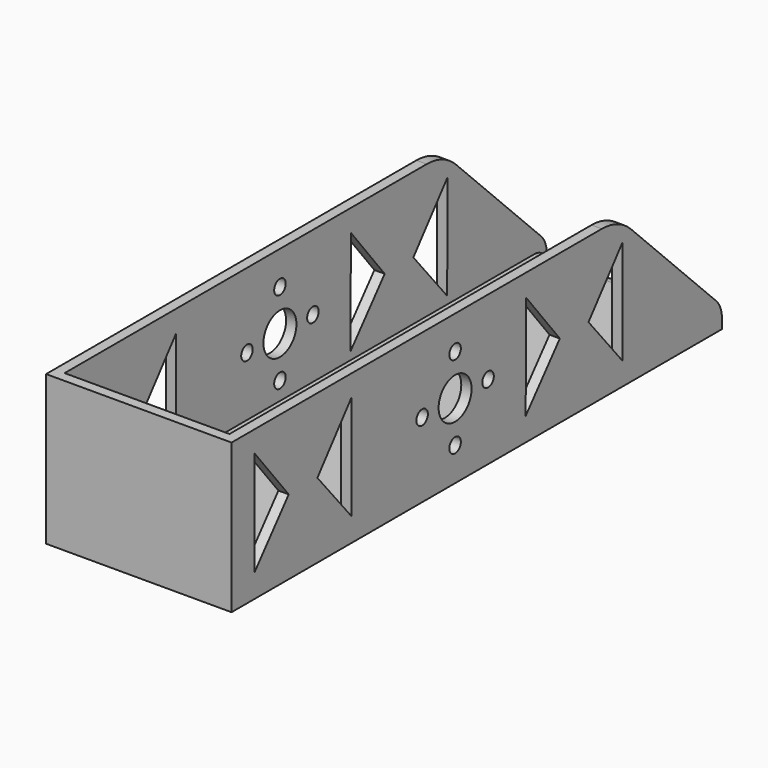
from build123d import *

# Parameters (mm, degrees)
F0_W      = 36
F0_H      = 119
F1_DEPTH  = 3
F3_DEPTH  = 26
F5_SIZE   = 25
F6_R      = 10
F7_R      = 2.99999
F8_R      = 5
F10_DEPTH = 25
F9_R      = 1.4
F9_R_2    = 4
F11_DEPTH = 36.001


# Not quite as in the source:
# - a fillet or chamfer is up to 0.001 mm smaller than in the source, because OpenCascade refuses the exact size


with BuildPart() as f1:
    # F0 (on Top) → F1 (new body)
    with BuildSketch(Plane.XY):
        Rectangle(F0_W, F0_H)
    extrude(amount=F1_DEPTH)

    # F2 (on face) → F3 (join)
    with BuildSketch(Plane.XY.offset(3)):
        Polygon((16, -57.5), (-16, -57.5), (-16, 57.5), (-16, 59.5), (-18, 59.5), (-18, -59.5), (18, -59.5), (18, 59.5), (16, 59.5), (16, 57.5), align=None)
    extrude(amount=F3_DEPTH)

    # F5
    f5_edges = [f1.edges().sort_by_distance(p)[0] for p in [
        (-17, 59.5, 29),
        (17, 59.5, 29),
    ]]
    chamfer(f5_edges, length=F5_SIZE)

    # F6
    f6_edges = [f1.edges().sort_by_distance(p)[0] for p in [
        (17, 34.5, 29),
        (-17, 34.5, 29),
    ]]
    fillet(f6_edges, radius=F6_R)

    # F7 (radius 3 in the source; OpenCascade refuses exactly that, so slightly less here)
    f7_edges = [f1.edges().sort_by_distance(p)[0] for p in [
        (0, 59.5, 3),
    ]]
    fillet(f7_edges, radius=F7_R)

    # F8
    f8_edges = [f1.edges().sort_by_distance(p)[0] for p in [
        (17, 59.5, 4),
        (-17, 59.5, 4),
    ]]
    fillet(f8_edges, radius=F8_R)

    # F4 (on face) → F10 (cut)
    with BuildSketch(Plane.XY.offset(3)):
        with BuildLine():
            ThreePointArc((-1.2459935794, 48.5), (-1.95, 47), (-1.2459935794, 45.5))
            ThreePointArc((-1.2459935794, 45.5), (0, 45.05), (1.2459935794, 45.5))
            ThreePointArc((1.2459935794, 45.5), (1.7652460848, 46.1715036149), (1.95, 47))
            ThreePointArc((1.95, 47), (1.7652460848, 47.8284963851), (1.2459935794, 48.5))
            ThreePointArc((1.2459935794, 48.5), (0, 48.95), (-1.2459935794, 48.5))
        make_face()
    extrude(amount=-F10_DEPTH, mode=Mode.SUBTRACT)

    # F9 (on face) → F11 (cut, through all)
    with BuildSketch(Plane.YZ.offset(18)):
        with Locations((-5.25, 22.5)):
            Circle(F9_R)
        with Locations((2.75, 14.5)):
            Circle(F9_R)
        with Locations((-5.25, 14.5)):
            Circle(F9_R_2)
        with Locations((-5.25, 6.5)):
            Circle(F9_R)
        with Locations((-13.25, 14.5)):
            Circle(F9_R)
        Polygon((-45.6205420196, 14.5), (-53.8677945733, 24.8276256025), (-53.8677945733, 4.6137683094), align=None)
        Polygon((-30.4197221994, 24.8276256025), (-38.6669747531, 14.5), (-30.4197221994, 4.6137683094), align=None)
        Polygon((11.8845089816, 4.5387393932), (20.1667771096, 14.395655056), (11.9562095653, 24.7524695214), align=None)
        Polygon((35.4041344278, 24.6692968517), (27.1203006313, 14.3709900539), (35.3324338441, 4.4555667236), align=None)
    extrude(amount=-F11_DEPTH, mode=Mode.SUBTRACT)


solid = f1.part
